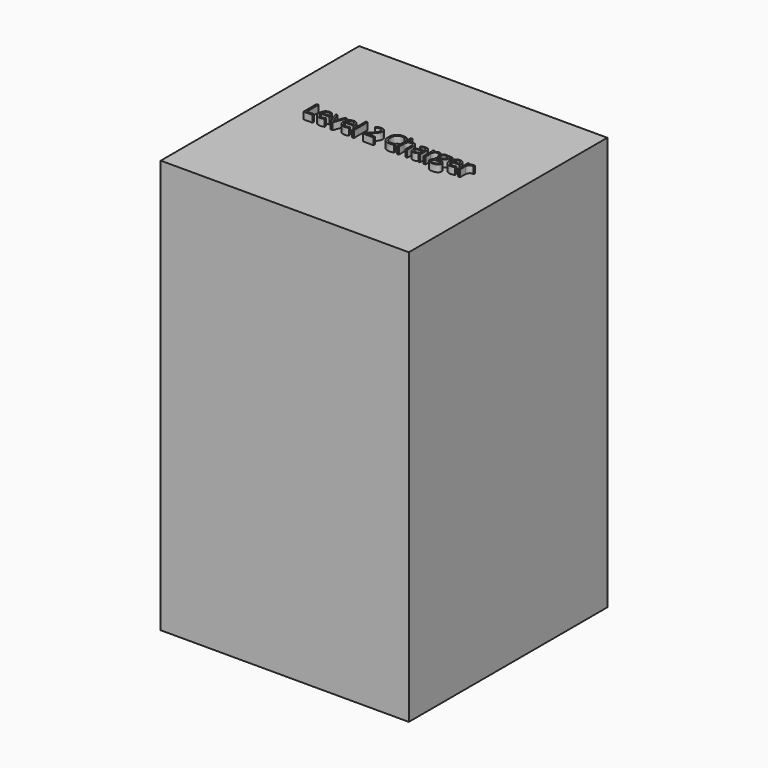
from build123d import *

# Parameters (mm, degrees)
F0_W         = 914.4
F0_H         = 914.4
F1_DEPTH     = 1524
F2_TEXT_SIZE = 83.9272038893
F3_DEPTH     = 25.4


# Not quite as in the source:
# - Text() gives the source's letters only with a copy of the font that has no kerning and outlines rounded to 1/6400 em; it was checked with that copy


with BuildPart() as f1:
    # F0 (on Top) → F1 (new body)
    with BuildSketch(Plane.XY):
        Rectangle(F0_W, F0_H)
    extrude(amount=F1_DEPTH)

    # F2 (on face) → F3 (join)
    with BuildSketch(Plane.XY.offset(1524)):
        with Locations((-304.8, 0)):
            Text('Level 2 Charger', F2_TEXT_SIZE, font='Open Sans', text_align=(TextAlign.LEFT, TextAlign.BOTTOM))
    extrude(amount=F3_DEPTH)


solid = f1.part
